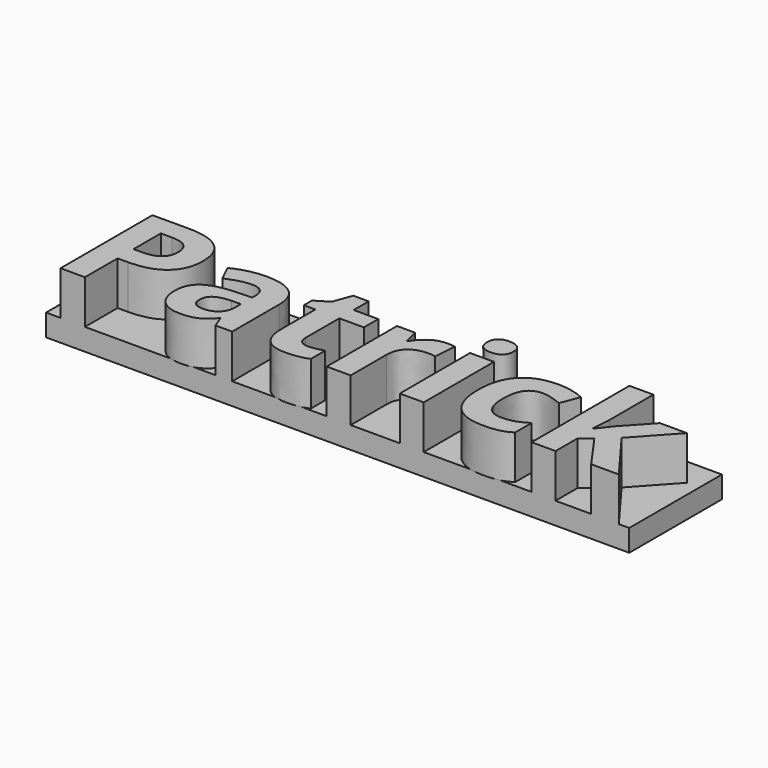
from build123d import *

# Parameters (mm, degrees)
F1_W         = 80
F1_H         = 15.8917101349
F2_DEPTH     = 3
F0_TEXT_SIZE = 22.0718196318
F3_DEPTH     = 6


# Not quite as in the source:
# - Text() gives the source's letters only with a copy of the font that has no kerning and outlines rounded to 1/6400 em; it was checked with that copy


with BuildPart() as f2:
    # F1 (on Top) → F2 (new body)
    with BuildSketch(Plane.XY):
        with Locations((24.8624477718, 0.2717083744)):
            Rectangle(F1_W, F1_H)
    extrude(amount=-F2_DEPTH)

    # F0 (on Top) → F3 (join)
    with BuildSketch(Plane.XY):
        with Locations((-15.1375522282, -7.6741466931)):
            Text('Patrick', F0_TEXT_SIZE, font='Open Sans', font_style=FontStyle.BOLD, text_align=(TextAlign.LEFT, TextAlign.BOTTOM))
    extrude(amount=F3_DEPTH)


solid = f2.part
